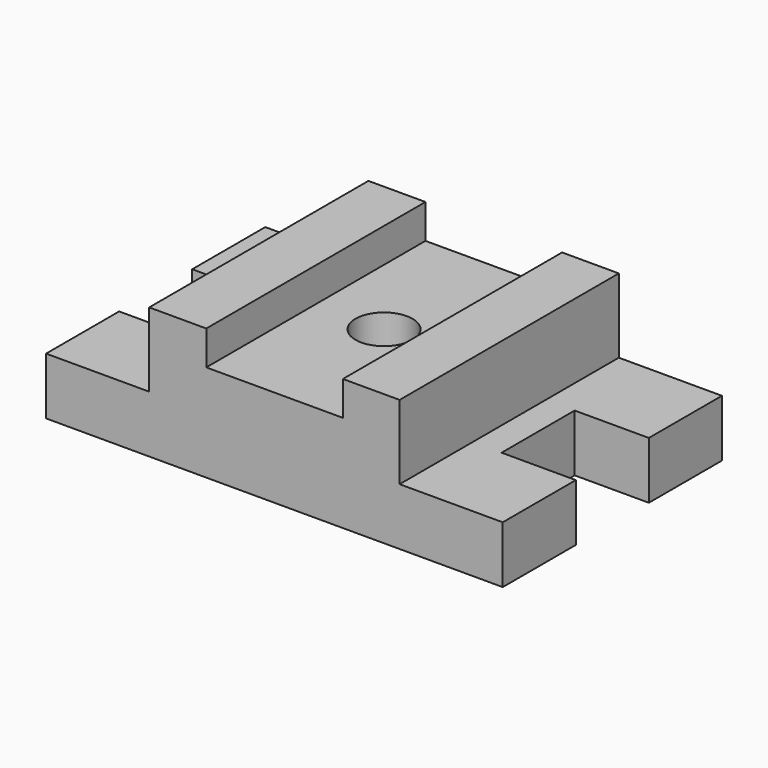
from build123d import *

# Parameters (mm, degrees)
F1_DEPTH  = 31.75
F2_W      = 69.6489959955
F2_H      = 152.4
F3_DEPTH  = 22.225
F4_W      = 31.5489959955
F4_H      = 152.4
F5_DEPTH  = 19.05
F6_W      = 31.5489959955
F6_H      = 31.75
F7_DEPTH  = 19.05
F9_D      = 31.75
F10_DEPTH = 19.05
F11_DEPTH = 19.05
F12_DEPTH = 19.05


# Not quite as in the source:
# - a feature names something its author has since deleted; it is built from what else it names


with BuildPart() as f1:
    # F0 (on Top) → F1 (new body)
    with BuildSketch(Plane.XY):
        Polygon((0, -76.2), (0, 76.2), (-127, 76.2), (-127, 25.4), (-85.725, 25.4), (-85.725, -25.4), (-127, -25.4), (-127, -76.2), align=None)
        Polygon((127, 25.4), (127, 76.2), (0, 76.2), (0, -76.2), (127, -76.2), (127, -25.4), (85.725, -25.4), (85.725, 25.4), align=None)
    extrude(amount=F1_DEPTH)

    # F2 (on face) → F3 (join)
    with BuildSketch(Plane.XY.offset(31.75)):
        with Locations((34.8244979978, 0)):
            Rectangle(F2_W, F2_H)
        with Locations((-34.8244979978, 0)):
            Rectangle(F2_W, F2_H)
    extrude(amount=F3_DEPTH)

    # F4 (on face) → F5 (join)
    with BuildSketch(Plane.XY.offset(53.975)):
        with Locations((53.8744979978, 0)):
            Rectangle(F4_W, F4_H)
    extrude(amount=F5_DEPTH)

    # F6 (on face) → F7 (join)
    with BuildSketch(Plane.XY):
        with Locations((53.8744979978, -60.325)):
            Rectangle(F6_W, F6_H)
        with Locations((-53.8744979978, -60.325)):
            Rectangle(F6_W, F6_H)
        with Locations((-53.8744979978, 60.325)):
            Rectangle(F6_W, F6_H)
        with Locations((53.8744979978, 60.325)):
            Rectangle(F6_W, F6_H)
    extrude(amount=F7_DEPTH)

    # F9 (through all)
    with Locations(Plane.XY.offset(53.975)):
        with Locations((0, 0)):
            Hole(F9_D / 2)

    # F6 (on face) → F10 (join)
    with BuildSketch(Plane.XY):
        with Locations((53.8744979978, 60.325)):
            Rectangle(F6_W, F6_H)
        with Locations((-53.8744979978, 60.325)):
            Rectangle(F6_W, F6_H)
        with Locations((-53.8744979978, -60.325)):
            Rectangle(F6_W, F6_H)
        with Locations((53.8744979978, -60.325)):
            Rectangle(F6_W, F6_H)
    extrude(amount=F10_DEPTH)

    # F4 (on face) → F11 (join)
    with BuildSketch(Plane.XY.offset(53.975)):
        with Locations((53.8744979978, 0)):
            Rectangle(F4_W, F4_H)
    extrude(amount=F11_DEPTH)

    # F4 (on face) → F12 (join)
    with BuildSketch(Plane.XY.offset(53.975)):
        Polygon((-37.8989959955, -76.2), (-37.8989959955, 76.2), (-69.6489959955, 76.2), (-69.6489959955, -76.2), (-38.1, -76.2), align=None)
    extrude(amount=F12_DEPTH)


solid = f1.part
